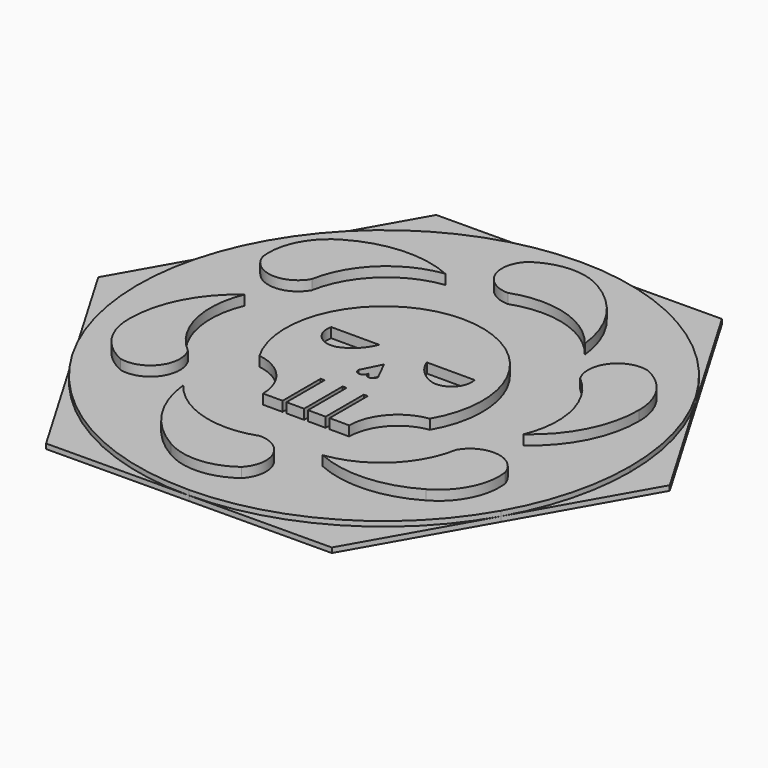
from build123d import *

# Parameters (mm, degrees)
F1_DEPTH = 1
F2_DEPTH = 0.5
F3_DEPTH = 0.25


# Not quite as in the source:
# - ends of sketch curves that miss each other by under 0.0002 mm in the source are joined


with BuildPart() as f1:
    # F0 (on Top) → F1 (new body)
    with BuildSketch(Plane.XY):
        with BuildLine():
            Line((0, 10.9258579865), (0, 7.8724477552))
            ThreePointArc((0, 7.8724477552), (2.7950316712, 7.9576349039), (5.1007339242, 6.3754857283))
            ThreePointArc((5.1007339242, 6.3754857283), (4.2373266186, 8.8147505289), (2.3540830685, 10.5892585378))
            ThreePointArc((2.3540830685, 10.5892585378), (1.2106007472, 10.992262078), (0, 10.9258579865))
        make_face()
        with BuildLine():
            ThreePointArc((-1.0926483052, 10.4001245921), (-1.3768651451, 8.7772651175), (0, 7.8724477552))
            Line((0, 7.8724477552), (0, 10.9258579865))
            ThreePointArc((0, 10.9258579865), (-0.5722795066, 10.7169351207), (-1.0926483052, 10.4001245921))
        make_face()
    extrude(amount=F1_DEPTH)


with BuildPart() as f1b:
    # F0 (on Top) → F1, piece 2 (new body)
    with BuildSketch(Plane.XY):
        with BuildLine():
            ThreePointArc((-6.817739746, 3.9362238776), (-5.4939981452, 6.3993858836), (-2.97096564, 7.6051080205))
            ThreePointArc((-2.97096564, 7.6051080205), (-5.5151345767, 8.0770077603), (-7.9935253667, 7.3333250088))
            ThreePointArc((-7.9935253667, 7.3333250088), (-9.2415971043, 6.0307184409), (-9.5530962519, 4.2538011064))
            ThreePointArc((-9.5530962519, 4.2538011064), (-8.28976714, 3.1962323655), (-6.817739746, 3.9362238776))
        make_face()
    extrude(amount=F1_DEPTH)


with BuildPart() as f1c:
    # F0 (on Top) → F1, piece 3 (new body)
    with BuildSketch(Plane.XY):
        with BuildLine():
            ThreePointArc((-6.817739746, -3.9362238776), (-8.2890298165, -1.5582490203), (-8.0716995643, 1.2296222922))
            ThreePointArc((-8.0716995643, 1.2296222922), (-9.7524611953, -0.7377427686), (-10.3476084352, -3.255933529))
            ThreePointArc((-10.3476084352, -3.255933529), (-9.843553925, -4.9880986434), (-8.4604479467, -6.1463234858))
            ThreePointArc((-8.4604479467, -6.1463234858), (-6.9129019949, -5.5810327519), (-6.817739746, -3.9362238776))
        make_face()
    extrude(amount=F1_DEPTH)


with BuildPart() as f1d:
    # F0 (on Top) → F1, piece 4 (new body)
    with BuildSketch(Plane.XY):
        with BuildLine():
            ThreePointArc((0, -7.8724477552), (-2.7950316712, -7.9576349039), (-5.1007339242, -6.3754857283))
            ThreePointArc((-5.1007339242, -6.3754857283), (-4.2373266186, -8.8147505289), (-2.3540830685, -10.5892585378))
            ThreePointArc((-2.3540830685, -10.5892585378), (-0.6019568208, -11.0188170843), (1.0926483052, -10.4001245921))
            ThreePointArc((1.0926483052, -10.4001245921), (1.3768651451, -8.7772651175), (0, -7.8724477552))
        make_face()
    extrude(amount=F1_DEPTH)


with BuildPart() as f1e:
    # F0 (on Top) → F1, piece 5 (new body)
    with BuildSketch(Plane.XY):
        with BuildLine():
            ThreePointArc((6.817739746, -3.9362238776), (5.4939981452, -6.3993858836), (2.97096564, -7.6051080205))
            ThreePointArc((2.97096564, -7.6051080205), (5.5151345767, -8.0770077603), (7.9935253667, -7.3333250088))
            ThreePointArc((7.9935253667, -7.3333250088), (9.2415971043, -6.0307184409), (9.5530962519, -4.2538011064))
            ThreePointArc((9.5530962519, -4.2538011064), (8.28976714, -3.1962323655), (6.817739746, -3.9362238776))
        make_face()
    extrude(amount=F1_DEPTH)


with BuildPart() as f1f:
    # F0 (on Top) → F1, piece 6 (new body)
    with BuildSketch(Plane.XY):
        with BuildLine():
            ThreePointArc((6.817739746, 3.9362238776), (8.2890298165, 1.5582490203), (8.0716995643, -1.2296222922))
            ThreePointArc((8.0716995643, -1.2296222922), (9.7524611953, 0.7377427686), (10.3476084352, 3.255933529))
            ThreePointArc((10.3476084352, 3.255933529), (9.843553925, 4.9880986434), (8.4604479467, 6.1463234858))
            ThreePointArc((8.4604479467, 6.1463234858), (6.9129019949, 5.5810327519), (6.817739746, 3.9362238776))
        make_face()
    extrude(amount=F1_DEPTH)


with BuildPart() as f1g:
    # F0 (on Top) → F1, piece 7 (new body)
    with BuildSketch(Plane.XY):
        with BuildLine():
            ThreePointArc((2.1873986951, -4.9489795918), (2.8057790938, -3.3281528305), (4.3301270189, -2.5))
            ThreePointArc((4.3301270189, -2.5), (4.3301270189, 2.5), (0, 5))
            Line((0, 5), (0, 1.2))
            Line((0, 1.2), (0, 0))
            Line((0, 0), (0.5, -1))
            ThreePointArc((0.5, -1), (0.25, -1.25), (0, -1))
            Line((0, -1), (0, -1.5))
            Line((0, -1.5), (0, -2.5))
            Line((0, -2.5), (0.1, -2.5000082476))
            Line((0.1, -2.5000082476), (0.1, -4.7830082476))
            Line((0.1, -4.7830082476), (0.1, -4.9489795918))
            Line((0.1, -4.9489795918), (0.9936993476, -4.9489795918))
            Line((0.9936993476, -4.9489795918), (0.9936993476, -4.8104380257))
            Line((0.9936993476, -4.8104380257), (0.9936993476, -2.5274380257))
            Line((0.9936993476, -2.5274380257), (1.1936993476, -2.5274380257))
            Line((1.1936993476, -2.5274380257), (1.1936993476, -4.8104380257))
            Line((1.1936993476, -4.8104380257), (1.1936993476, -4.9489795918))
            Line((1.1936993476, -4.9489795918), (2.1873986951, -4.9489795918))
        make_face()
        with BuildLine():
            ThreePointArc((2.4269322199, 0), (1.6857796426, 0.4640720542), (1.21346611, 1.2))
            Line((1.21346611, 1.2), (2.4269322199, 1.2))
            Line((2.4269322199, 1.2), (3.6403983299, 1.2))
            ThreePointArc((3.6403983299, 1.2), (3.370181606, 0.2597073639), (2.4269322199, 0))
        make_face(mode=Mode.SUBTRACT)
        with BuildLine():
            Line((0, 1.2), (0, 5))
            ThreePointArc((0, 5), (-4.3301270189, 2.5), (-4.3301270189, -2.5))
            ThreePointArc((-4.3301270189, -2.5), (-2.8057790938, -3.3281528305), (-2.1873986951, -4.9489795918))
            Line((-2.1873986951, -4.9489795918), (-1.1936993476, -4.9489795918))
            Line((-1.1936993476, -4.9489795918), (-1.1936993476, -4.8104380257))
            Line((-1.1936993476, -4.8104380257), (-1.1936993476, -2.5274380257))
            Line((-1.1936993476, -2.5274380257), (-0.9936993476, -2.5274380257))
            Line((-0.9936993476, -2.5274380257), (-0.9936993476, -4.8104380257))
            Line((-0.9936993476, -4.8104380257), (-0.9936993476, -4.9489795918))
            Line((-0.9936993476, -4.9489795918), (-0.1, -4.9489795918))
            Line((-0.1, -4.9489795918), (-0.1, -4.7830082476))
            Line((-0.1, -4.7830082476), (-0.1, -2.5000082476))
            Line((-0.1, -2.5000082476), (0, -2.5000082476))
            Line((0, -2.5000082476), (0, -1.5))
            Line((0, -1.5), (0, -1))
            ThreePointArc((0, -1), (-0.25, -1.25), (-0.5, -1))
            Line((-0.5, -1), (0, 0))
            Line((0, 0), (0, 1.2))
        make_face()
        with BuildLine():
            Line((-2.4269322199, 1.2), (-1.21346611, 1.2))
            ThreePointArc((-1.21346611, 1.2), (-1.6857796426, 0.4640720542), (-2.4269322199, 0))
            ThreePointArc((-2.4269322199, 0), (-3.370181606, 0.2597073639), (-3.6403983299, 1.2))
            Line((-3.6403983299, 1.2), (-2.4269322199, 1.2))
        make_face(mode=Mode.SUBTRACT)
    extrude(amount=F1_DEPTH)


with BuildPart() as f2:
    # F0 (on Top) → F2 (new body)
    with BuildSketch(Plane.XY):
        with BuildLine():
            ThreePointArc((10.7800154824, 6.3278168588), (6.2109697015, 10.8477580802), (0, 12.5))
            ThreePointArc((0, 12.5), (-0.0450215705, 12.4999189221), (-0.090042557, 12.4996756893))
            ThreePointArc((-0.090042557, 12.4996756893), (-6.3278168731, 10.7800154741), (-10.8700578347, 6.1718589315))
            ThreePointArc((-10.8700578347, 6.1718589315), (-12.4996756914, -0.0900422734), (-10.7800155615, -6.3278167241))
            ThreePointArc((-10.7800155615, -6.3278167241), (-6.1718588351, -10.8700578894), (0.090042557, -12.4996756893))
            ThreePointArc((0.090042557, -12.4996756893), (6.3278168712, -10.7800154752), (10.8700578325, -6.1718589353))
            ThreePointArc((10.8700578325, -6.1718589353), (12.0856469191, -3.1917297108), (12.5, 0))
            ThreePointArc((12.5, 0), (12.0623420929, 3.2787045056), (10.7800154824, 6.3278168588))
        make_face()
        with BuildLine():
            ThreePointArc((-2.3540830685, -10.5892585378), (-4.2373266186, -8.8147505289), (-5.1007339242, -6.3754857283))
            ThreePointArc((-5.1007339242, -6.3754857283), (-2.7950316712, -7.9576349039), (0, -7.8724477552))
            ThreePointArc((0, -7.8724477552), (1.3768651451, -8.7772651175), (1.0926483052, -10.4001245921))
            ThreePointArc((1.0926483052, -10.4001245921), (-0.6019568208, -11.0188170843), (-2.3540830685, -10.5892585378))
        make_face(mode=Mode.SUBTRACT)
        with BuildLine():
            ThreePointArc((-10.3476084352, -3.255933529), (-9.7524611953, -0.7377427686), (-8.0716995643, 1.2296222922))
            ThreePointArc((-8.0716995643, 1.2296222922), (-8.2890298165, -1.5582490203), (-6.817739746, -3.9362238776))
            ThreePointArc((-6.817739746, -3.9362238776), (-6.9129019949, -5.5810327519), (-8.4604479467, -6.1463234858))
            ThreePointArc((-8.4604479467, -6.1463234858), (-9.843553925, -4.9880986434), (-10.3476084352, -3.255933529))
        make_face(mode=Mode.SUBTRACT)
        with BuildLine():
            ThreePointArc((7.9935253667, -7.3333250088), (5.5151345767, -8.0770077603), (2.97096564, -7.6051080205))
            ThreePointArc((2.97096564, -7.6051080205), (5.4939981452, -6.3993858836), (6.817739746, -3.9362238776))
            ThreePointArc((6.817739746, -3.9362238776), (8.28976714, -3.1962323655), (9.5530962519, -4.2538011064))
            ThreePointArc((9.5530962519, -4.2538011064), (9.2415971043, -6.0307184409), (7.9935253667, -7.3333250088))
        make_face(mode=Mode.SUBTRACT)
        with BuildLine():
            ThreePointArc((-7.9935253667, 7.3333250088), (-5.5151345767, 8.0770077603), (-2.97096564, 7.6051080205))
            ThreePointArc((-2.97096564, 7.6051080205), (-5.4939981452, 6.3993858836), (-6.817739746, 3.9362238776))
            ThreePointArc((-6.817739746, 3.9362238776), (-8.28976714, 3.1962323655), (-9.5530962519, 4.2538011064))
            ThreePointArc((-9.5530962519, 4.2538011064), (-9.2415971043, 6.0307184409), (-7.9935253667, 7.3333250088))
        make_face(mode=Mode.SUBTRACT)
        with BuildLine():
            ThreePointArc((0, 5), (4.3301270189, 2.5), (4.3301270189, -2.5))
            ThreePointArc((4.3301270189, -2.5), (2.8057790938, -3.3281528305), (2.1873986951, -4.9489795918))
            Line((2.1873986951, -4.9489795918), (1.1936993476, -4.9489795918))
            Line((1.1936993476, -4.9489795918), (0.9936993476, -4.9489795918))
            Line((0.9936993476, -4.9489795918), (0.1, -4.9489795918))
            Line((0.1, -4.9489795918), (0, -4.9489795918))
            Line((0, -4.9489795918), (-0.1, -4.9489795918))
            Line((-0.1, -4.9489795918), (-0.9936993476, -4.9489795918))
            Line((-0.9936993476, -4.9489795918), (-1.1936993476, -4.9489795918))
            Line((-1.1936993476, -4.9489795918), (-2.1873986951, -4.9489795918))
            ThreePointArc((-2.1873986951, -4.9489795918), (-2.8057790938, -3.3281528305), (-4.3301270189, -2.5))
            ThreePointArc((-4.3301270189, -2.5), (-4.3301270189, 2.5), (0, 5))
        make_face(mode=Mode.SUBTRACT)
        with BuildLine():
            ThreePointArc((10.3476084352, 3.255933529), (9.7524611953, 0.7377427686), (8.0716995643, -1.2296222922))
            ThreePointArc((8.0716995643, -1.2296222922), (8.2890298165, 1.5582490203), (6.817739746, 3.9362238776))
            ThreePointArc((6.817739746, 3.9362238776), (6.9129019949, 5.5810327519), (8.4604479467, 6.1463234858))
            ThreePointArc((8.4604479467, 6.1463234858), (9.843553925, 4.9880986434), (10.3476084352, 3.255933529))
        make_face(mode=Mode.SUBTRACT)
        with BuildLine():
            ThreePointArc((5.1007339242, 6.3754857283), (2.7950316712, 7.9576349039), (0, 7.8724477552))
            ThreePointArc((0, 7.8724477552), (-1.3768651451, 8.7772651175), (-1.0926483052, 10.4001245921))
            ThreePointArc((-1.0926483052, 10.4001245921), (-0.5722795066, 10.7169351207), (0, 10.9258579865))
            ThreePointArc((0, 10.9258579865), (1.2106007472, 10.992262078), (2.3540830685, 10.5892585378))
            ThreePointArc((2.3540830685, 10.5892585378), (4.2373266186, 8.8147505289), (5.1007339242, 6.3754857283))
        make_face(mode=Mode.SUBTRACT)
        Polygon((-1.1936993476, -4.8104380257), (-1.1936993476, -4.9489795918), (-0.9936993476, -4.9489795918), (-0.9936993476, -4.8104380257), (-0.9936993476, -2.5274380257), (-1.1936993476, -2.5274380257), align=None)
        Polygon((0, -4.9489795918), (0.1, -4.9489795918), (0.1, -4.7830082476), (0.1, -2.5000082476), (0, -2.5000082476), (-0.1, -2.5000082476), (-0.1, -4.7830082476), (-0.1, -4.9489795918), align=None)
        Polygon((0.9936993476, -4.9489795918), (1.1936993476, -4.9489795918), (1.1936993476, -4.8104380257), (1.1936993476, -2.5274380257), (0.9936993476, -2.5274380257), (0.9936993476, -4.8104380257), align=None)
    extrude(amount=F2_DEPTH)


with BuildPart() as f2b:
    # F0 (on Top) → F2, piece 2 (new body)
    with BuildSketch(Plane.XY):
        with BuildLine():
            ThreePointArc((-2.4269322199, 0), (-1.6857796426, 0.4640720542), (-1.21346611, 1.2))
            Line((-1.21346611, 1.2), (-2.4269322199, 1.2))
            Line((-2.4269322199, 1.2), (-3.6403983299, 1.2))
            ThreePointArc((-3.6403983299, 1.2), (-3.370181606, 0.2597073639), (-2.4269322199, 0))
        make_face()
    extrude(amount=F2_DEPTH)


with BuildPart() as f2c:
    # F0 (on Top) → F2, piece 3 (new body)
    with BuildSketch(Plane.XY):
        with BuildLine():
            Line((2.4269322199, 1.2), (1.21346611, 1.2))
            ThreePointArc((1.21346611, 1.2), (1.6857796426, 0.4640720542), (2.4269322199, 0))
            ThreePointArc((2.4269322199, 0), (3.370181606, 0.2597073639), (3.6403983299, 1.2))
            Line((3.6403983299, 1.2), (2.4269322199, 1.2))
        make_face()
    extrude(amount=F2_DEPTH)


with BuildPart() as f2d:
    # F0 (on Top) → F2, piece 4 (new body)
    with BuildSketch(Plane.XY):
        with BuildLine():
            Line((0.5, -1), (0, 0))
            Line((0, 0), (-0.5, -1))
            ThreePointArc((-0.5, -1), (-0.25, -1.25), (0, -1))
            ThreePointArc((0, -1), (0.25, -1.25), (0.5, -1))
        make_face()
    extrude(amount=F2_DEPTH)


with BuildPart() as f3:
    # F0 (on Top) → F3 (new body)
    with BuildSketch(Plane.XY):
        with BuildLine():
            ThreePointArc((10.7800154824, 6.3278168588), (6.2109697015, 10.8477580802), (0, 12.5))
            ThreePointArc((0, 12.5), (-0.0450215705, 12.4999189221), (-0.090042557, 12.4996756893))
            ThreePointArc((-0.090042557, 12.4996756893), (-6.3278168731, 10.7800154741), (-10.8700578347, 6.1718589315))
            ThreePointArc((-10.8700578347, 6.1718589315), (-12.4996756914, -0.0900422734), (-10.7800155615, -6.3278167241))
            ThreePointArc((-10.7800155615, -6.3278167241), (-6.1718588351, -10.8700578894), (0.090042557, -12.4996756893))
            ThreePointArc((0.090042557, -12.4996756893), (6.3278168712, -10.7800154752), (10.8700578325, -6.1718589353))
            ThreePointArc((10.8700578325, -6.1718589353), (12.0856469191, -3.1917297108), (12.5, 0))
            ThreePointArc((12.5, 0), (12.0623420929, 3.2787045056), (10.7800154824, 6.3278168588))
        make_face()
        with BuildLine():
            ThreePointArc((-2.3540830685, -10.5892585378), (-4.2373266186, -8.8147505289), (-5.1007339242, -6.3754857283))
            ThreePointArc((-5.1007339242, -6.3754857283), (-2.7950316712, -7.9576349039), (0, -7.8724477552))
            ThreePointArc((0, -7.8724477552), (1.3768651451, -8.7772651175), (1.0926483052, -10.4001245921))
            ThreePointArc((1.0926483052, -10.4001245921), (-0.6019568208, -11.0188170843), (-2.3540830685, -10.5892585378))
        make_face(mode=Mode.SUBTRACT)
        with BuildLine():
            ThreePointArc((-10.3476084352, -3.255933529), (-9.7524611953, -0.7377427686), (-8.0716995643, 1.2296222922))
            ThreePointArc((-8.0716995643, 1.2296222922), (-8.2890298165, -1.5582490203), (-6.817739746, -3.9362238776))
            ThreePointArc((-6.817739746, -3.9362238776), (-6.9129019949, -5.5810327519), (-8.4604479467, -6.1463234858))
            ThreePointArc((-8.4604479467, -6.1463234858), (-9.843553925, -4.9880986434), (-10.3476084352, -3.255933529))
        make_face(mode=Mode.SUBTRACT)
        with BuildLine():
            ThreePointArc((7.9935253667, -7.3333250088), (5.5151345767, -8.0770077603), (2.97096564, -7.6051080205))
            ThreePointArc((2.97096564, -7.6051080205), (5.4939981452, -6.3993858836), (6.817739746, -3.9362238776))
            ThreePointArc((6.817739746, -3.9362238776), (8.28976714, -3.1962323655), (9.5530962519, -4.2538011064))
            ThreePointArc((9.5530962519, -4.2538011064), (9.2415971043, -6.0307184409), (7.9935253667, -7.3333250088))
        make_face(mode=Mode.SUBTRACT)
        with BuildLine():
            ThreePointArc((-7.9935253667, 7.3333250088), (-5.5151345767, 8.0770077603), (-2.97096564, 7.6051080205))
            ThreePointArc((-2.97096564, 7.6051080205), (-5.4939981452, 6.3993858836), (-6.817739746, 3.9362238776))
            ThreePointArc((-6.817739746, 3.9362238776), (-8.28976714, 3.1962323655), (-9.5530962519, 4.2538011064))
            ThreePointArc((-9.5530962519, 4.2538011064), (-9.2415971043, 6.0307184409), (-7.9935253667, 7.3333250088))
        make_face(mode=Mode.SUBTRACT)
        with BuildLine():
            ThreePointArc((0, 5), (4.3301270189, 2.5), (4.3301270189, -2.5))
            ThreePointArc((4.3301270189, -2.5), (2.8057790938, -3.3281528305), (2.1873986951, -4.9489795918))
            Line((2.1873986951, -4.9489795918), (1.1936993476, -4.9489795918))
            Line((1.1936993476, -4.9489795918), (0.9936993476, -4.9489795918))
            Line((0.9936993476, -4.9489795918), (0.1, -4.9489795918))
            Line((0.1, -4.9489795918), (0, -4.9489795918))
            Line((0, -4.9489795918), (-0.1, -4.9489795918))
            Line((-0.1, -4.9489795918), (-0.9936993476, -4.9489795918))
            Line((-0.9936993476, -4.9489795918), (-1.1936993476, -4.9489795918))
            Line((-1.1936993476, -4.9489795918), (-2.1873986951, -4.9489795918))
            ThreePointArc((-2.1873986951, -4.9489795918), (-2.8057790938, -3.3281528305), (-4.3301270189, -2.5))
            ThreePointArc((-4.3301270189, -2.5), (-4.3301270189, 2.5), (0, 5))
        make_face(mode=Mode.SUBTRACT)
        with BuildLine():
            ThreePointArc((10.3476084352, 3.255933529), (9.7524611953, 0.7377427686), (8.0716995643, -1.2296222922))
            ThreePointArc((8.0716995643, -1.2296222922), (8.2890298165, 1.5582490203), (6.817739746, 3.9362238776))
            ThreePointArc((6.817739746, 3.9362238776), (6.9129019949, 5.5810327519), (8.4604479467, 6.1463234858))
            ThreePointArc((8.4604479467, 6.1463234858), (9.843553925, 4.9880986434), (10.3476084352, 3.255933529))
        make_face(mode=Mode.SUBTRACT)
        with BuildLine():
            ThreePointArc((5.1007339242, 6.3754857283), (2.7950316712, 7.9576349039), (0, 7.8724477552))
            ThreePointArc((0, 7.8724477552), (-1.3768651451, 8.7772651175), (-1.0926483052, 10.4001245921))
            ThreePointArc((-1.0926483052, 10.4001245921), (-0.5722795066, 10.7169351207), (0, 10.9258579865))
            ThreePointArc((0, 10.9258579865), (1.2106007472, 10.992262078), (2.3540830685, 10.5892585378))
            ThreePointArc((2.3540830685, 10.5892585378), (4.2373266186, 8.8147505289), (5.1007339242, 6.3754857283))
        make_face(mode=Mode.SUBTRACT)
        with BuildLine():
            ThreePointArc((-0.090042557, 12.4996756893), (-0.0450215705, 12.4999189221), (0, 12.5))
            ThreePointArc((0, 12.5), (6.2109697015, 10.8477580802), (10.7800154824, 6.3278168588))
            Line((10.7800154824, 6.3278168588), (7.1266485769, 12.5516617782))
            Line((7.1266485769, 12.5516617782), (-0.090042557, 12.4996756893))
        make_face()
        with BuildLine():
            Line((14.4333822481, 0.1039721776), (10.7800154824, 6.3278168588))
            ThreePointArc((10.7800154824, 6.3278168588), (12.0623420929, 3.2787045056), (12.5, 0))
            ThreePointArc((12.5, 0), (12.0856469191, -3.1917297108), (10.8700578325, -6.1718589353))
            Line((10.8700578325, -6.1718589353), (14.4333822481, 0.1039721776))
        make_face()
        with BuildLine():
            ThreePointArc((-10.8700578347, 6.1718589315), (-6.3278168731, 10.7800154741), (-0.090042557, 12.4996756893))
            Line((-0.090042557, 12.4996756893), (-7.3067336712, 12.4476896006))
            Line((-7.3067336712, 12.4476896006), (-10.8700578347, 6.1718589315))
        make_face()
        with BuildLine():
            ThreePointArc((-10.7800155615, -6.3278167241), (-12.4996756914, -0.0900422734), (-10.8700578347, 6.1718589315))
            Line((-10.8700578347, 6.1718589315), (-14.4333822481, -0.1039721776))
            Line((-14.4333822481, -0.1039721776), (-10.7800155615, -6.3278167241))
        make_face()
        with BuildLine():
            Line((7.3067336712, -12.4476896006), (10.8700578325, -6.1718589353))
            ThreePointArc((10.8700578325, -6.1718589353), (6.3278168712, -10.7800154752), (0.090042557, -12.4996756893))
            Line((0.090042557, -12.4996756893), (7.3067336712, -12.4476896006))
        make_face()
        with BuildLine():
            ThreePointArc((0.090042557, -12.4996756893), (-6.1718588351, -10.8700578894), (-10.7800155615, -6.3278167241))
            Line((-10.7800155615, -6.3278167241), (-7.1266485769, -12.5516617782))
            Line((-7.1266485769, -12.5516617782), (0.090042557, -12.4996756893))
        make_face()
    extrude(amount=F3_DEPTH)


solid = Compound([f1.part, f1b.part, f1c.part, f1d.part, f1e.part, f1f.part, f1g.part, f2.part, f2b.part, f2c.part, f2d.part, f3.part])
